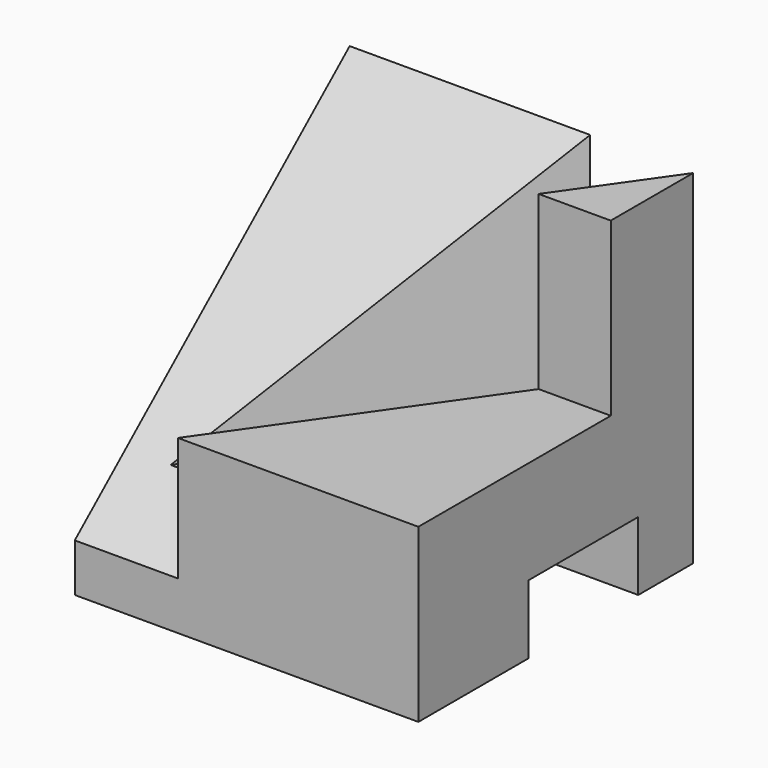
from build123d import *

# Parameters (mm, degrees)
F0_W     = 50
F0_H     = 50
F1_DEPTH = 50
F3_DEPTH = 35
F5_DEPTH = 25
F7_REACH = 115.9479483752
F8_W     = 20
F8_H     = 10
F9_DEPTH = 30


with BuildPart() as f1:
    # F0 (on Right) → F1 (new body)
    with BuildSketch(Plane.YZ):
        with Locations((25, 25)):
            Rectangle(F0_W, F0_H)
    extrude(amount=F1_DEPTH)

    # F2 (on face) → F3 (cut)
    with BuildSketch(Plane.XY.offset(50)):
        Polygon((0, 0), (15, 0), (50, 50), (35, 50), align=None)
    extrude(amount=-F3_DEPTH, mode=Mode.SUBTRACT)

    # F4 (on face) → F5 (cut)
    with BuildSketch(Plane.XY.offset(50)):
        Polygon((15, 0), (50, 0), (50, 35), (39.5, 35), align=None)
    extrude(amount=-F5_DEPTH, mode=Mode.SUBTRACT)

    f7_end = Plane(origin=(37.75, 32.5, 27.5), x_dir=(-0.5734623444, -0.8192319205, 0), z_dir=(-0.8192319205, 0.5734623444, 0))
    # F6 (on face) → F7 (cut, up to a plane its end follows)
    with BuildSketch(Plane(origin=(0, 0, 0), x_dir=(0, -1, 0), z_dir=(-1, 0, 0))):
        Polygon((-50, 50), (0, 7), (0, 15), (0, 50), align=None)
    f7_long = extrude(amount=-F7_REACH, mode=Mode.PRIVATE)
    add(split(f7_long, bisect_by=f7_end, keep=Keep.TOP, mode=Mode.PRIVATE), mode=Mode.SUBTRACT)

    # F8 (on face) → F9 (cut)
    with BuildSketch(Plane.YZ.offset(50)):
        with Locations((30, 5)):
            Rectangle(F8_W, F8_H)
    extrude(amount=-F9_DEPTH, mode=Mode.SUBTRACT)


solid = f1.part
